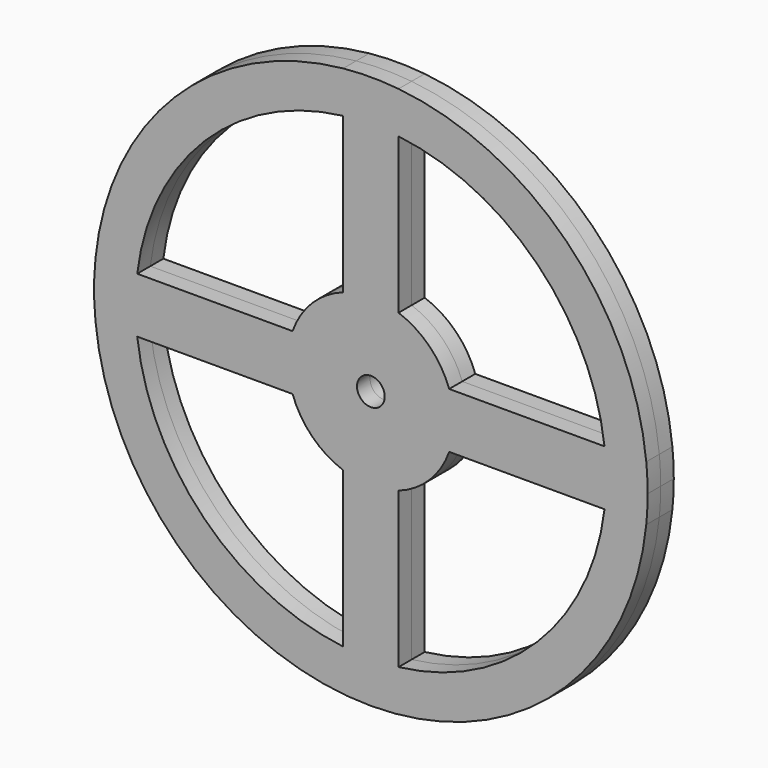
from build123d import *

# Parameters (mm, degrees)
F0_R     = 12.7
F1_DEPTH = 14.986


# Not quite as in the source:
# - a feature names something its author has since deleted; it is built from what else it names


with BuildPart() as f1:
    # F0 (on Front) → F1 (new body, symmetric)
    with BuildSketch(Plane.XZ):
        with BuildLine():
            ThreePointArc((252.7268090251, -25.4), (253.68150257, -12.7159448652), (254, 0))
            ThreePointArc((254, 0), (253.68150257, 12.7159448652), (252.7268090251, 25.4))
            ThreePointArc((252.7268090251, 25.4), (179.6051224214, 179.6051224214), (25.4, 252.7268090251))
            ThreePointArc((25.4, 252.7268090251), (0, 254), (-25.4, 252.7268090251))
            ThreePointArc((-25.4, 252.7268090251), (-179.6051224214, 179.6051224214), (-252.7268090251, 25.4))
            ThreePointArc((-252.7268090251, 25.4), (-254, 0), (-252.7268090251, -25.4))
            ThreePointArc((-252.7268090251, -25.4), (-179.6051224214, -179.6051224214), (-25.4, -252.7268090251))
            ThreePointArc((-25.4, -252.7268090251), (-1.543e-07, -254), (25.399999693, -252.7268090559))
            ThreePointArc((25.399999693, -252.7268090559), (179.6051223123, -179.6051225305), (252.7268090251, -25.4))
        make_face()
        with BuildLine():
            ThreePointArc((-25.4, -214.4006763049), (-152.6643540582, -152.6643540582), (-214.4006763049, -25.4))
            Line((-214.4006763049, -25.4), (-71.8420489686, -25.4))
            ThreePointArc((-71.8420489686, -25.4), (-53.8815367264, -53.8815367264), (-25.4, -71.8420489686))
            Line((-25.4, -71.8420489686), (-25.4, -214.4006763049))
        make_face(mode=Mode.SUBTRACT)
        with BuildLine():
            ThreePointArc((25.399999693, -71.8420490771), (53.8815366113, -53.8815368415), (71.8420489686, -25.4))
            Line((71.8420489686, -25.4), (214.4006763049, -25.4))
            ThreePointArc((214.4006763049, -25.4), (152.6643539489, -152.6643541675), (25.399999693, -214.4006763413))
            Line((25.399999693, -214.4006763413), (25.399999693, -71.8420490771))
        make_face(mode=Mode.SUBTRACT)
        with BuildLine():
            Line((-25.4, 214.4006763049), (-25.4, 71.8420489686))
            ThreePointArc((-25.4, 71.8420489686), (-53.8815367264, 53.8815367264), (-71.8420489686, 25.4))
            Line((-71.8420489686, 25.4), (-214.4006763049, 25.4))
            ThreePointArc((-214.4006763049, 25.4), (-152.6643540582, 152.6643540582), (-25.4, 214.4006763049))
        make_face(mode=Mode.SUBTRACT)
        Circle(F0_R, mode=Mode.SUBTRACT)
        with BuildLine():
            ThreePointArc((71.8420489686, 25.4), (53.8815367264, 53.8815367264), (25.4, 71.8420489686))
            Line((25.4, 71.8420489686), (25.4, 214.4006763049))
            ThreePointArc((25.4, 214.4006763049), (152.6643540582, 152.6643540582), (214.4006763049, 25.4))
            Line((214.4006763049, 25.4), (71.8420489686, 25.4))
        make_face(mode=Mode.SUBTRACT)
    extrude(amount=F1_DEPTH, both=True)


solid = f1.part
